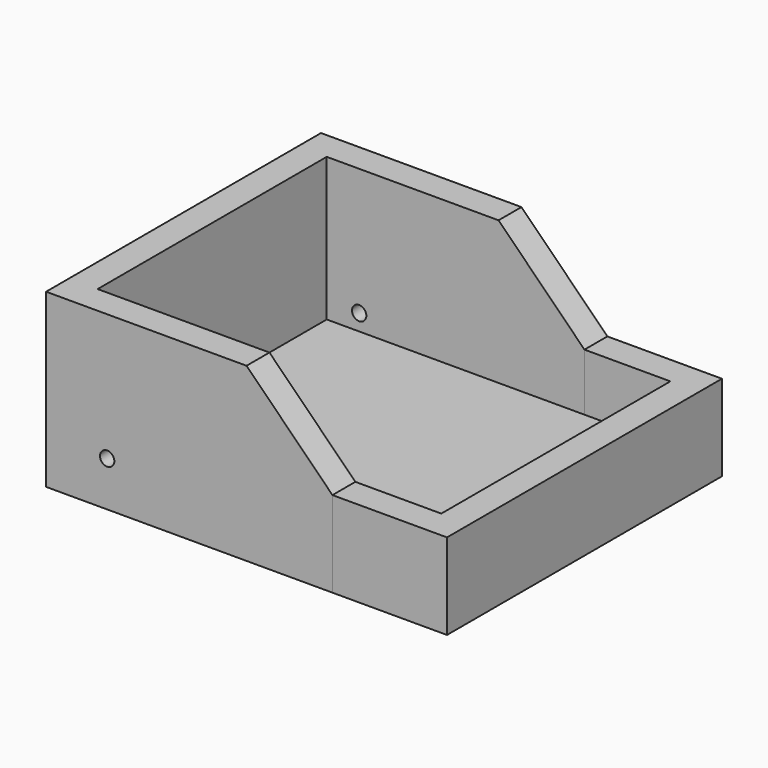
from build123d import *

# Parameters (mm, degrees)
F1_DEPTH = 76.2
F2_DEPTH = 38.1
F3_SIZE  = 38.1
F0_W     = 114.3
F0_H     = 127
F0_W_2   = 38.1
F4_DEPTH = 12.7
F6_D     = 6.35


with BuildPart() as f1:
    # F0 (on Top) → F1 (new body)
    with BuildSketch(Plane.XY):
        Polygon((-88.9, -76.2), (38.1, -76.2), (38.1, -63.5), (-76.2, -63.5), (-76.2, 63.5), (38.1, 63.5), (38.1, 76.2), (-88.9, 76.2), align=None)
    extrude(amount=F1_DEPTH)

    # F3
    f3_edges = [f1.edges().sort_by_distance(p)[0] for p in [
        (38.1, -69.85, 76.2),
        (38.1, 69.85, 76.2),
    ]]
    chamfer(f3_edges, length=F3_SIZE)

    # F0 (on Top) → F4 (join)
    with BuildSketch(Plane.XY):
        with Locations((-19.05, 0)):
            Rectangle(F0_W, F0_H)
        with Locations((57.15, 0)):
            Rectangle(F0_W_2, F0_H)
    extrude(amount=F4_DEPTH)

    # F6 (through all)
    with Locations(Plane(origin=(0, 76.2, 0), x_dir=(-1, 0, 0), z_dir=(0, 1, 0))):
        with Locations((61.8133324465, 19.8607390972)):
            Hole(F6_D / 2)


with BuildPart() as f2:
    # F0 (on Top) → F2 (new body)
    with BuildSketch(Plane.XY):
        Polygon((38.1, -76.2), (88.9, -76.2), (88.9, 76.2), (38.1, 76.2), (38.1, 63.5), (76.2, 63.5), (76.2, -63.5), (38.1, -63.5), align=None)
    extrude(amount=F2_DEPTH)


solid = Compound([f1.part, f2.part])
